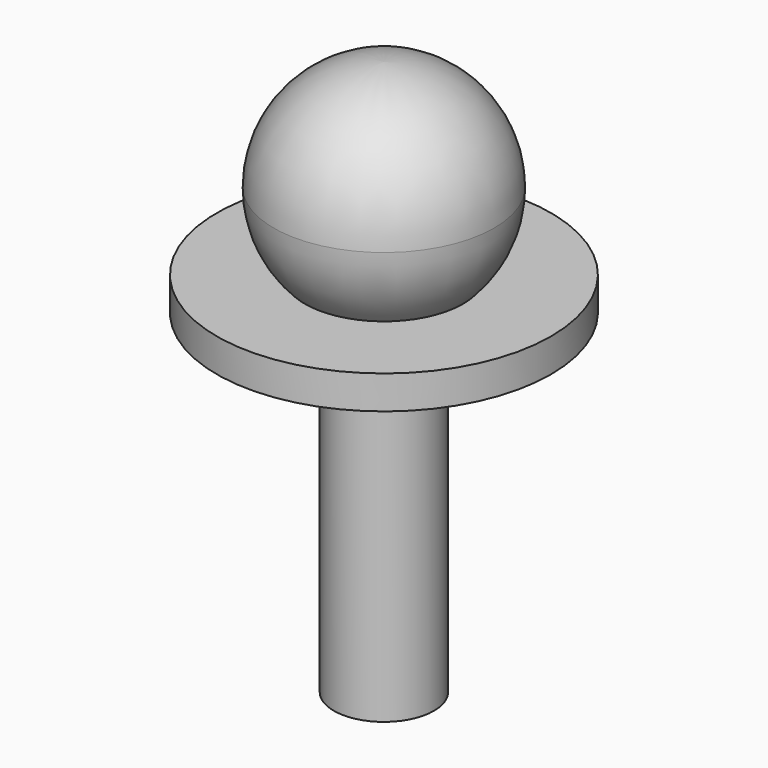
from build123d import *

# Parameters (mm, degrees)
F0_R      = 4.191
F1_DEPTH  = 73.66
F2_R      = 4.191
F3_DEPTH  = 8.382
F4_R      = 4.19099
F5_R      = 6.35
F6_DEPTH  = 1.27
F7_R      = 29.9024876922
F8_DEPTH  = 73.66
F9_R      = 1.905
F10_DEPTH = 12.7


# Not quite as in the source:
# - a fillet or chamfer is up to 0.001 mm smaller than in the source, because OpenCascade refuses the exact size


with BuildPart() as f1:
    # F0 (on Top) → F1 (new body)
    with BuildSketch(Plane.XY):
        Circle(F0_R)
    extrude(amount=F1_DEPTH)



with BuildPart() as f3:
    # F2 (on face) → F3 (new body)
    with BuildSketch(Plane.XY.offset(73.66)):
        Circle(F2_R)
    extrude(amount=F3_DEPTH)

    # F4 (radius 4.191 in the source; OpenCascade refuses exactly that, so slightly less here)
    f4_edges = [f3.edges().sort_by_distance(p)[0] for p in [
        (-4.191, 0, 73.66),
        (-4.191, 0, 82.042),
    ]]
    fillet(f4_edges, radius=F4_R)


with BuildPart() as f1_1:
    add(f1.part)

    add(f3.part)  # F6 merges F3
    # F5 (on face) → F6 (join)
    with BuildSketch(Plane.XY.offset(73.66)):
        Circle(F5_R)
    extrude(amount=F6_DEPTH)

    # F7 (on face) → F8 (cut)
    with BuildSketch(Plane(origin=(0, 0, 0), x_dir=(1, 0, 0), z_dir=(0, 0, -1))):
        Circle(F7_R)
    extrude(amount=-F8_DEPTH, mode=Mode.SUBTRACT)

    # F9 (on face) → F10 (join)
    with BuildSketch(Plane(origin=(0, 0, 73.66), x_dir=(1, 0, 0), z_dir=(0, 0, -1))):
        Circle(F9_R)
    extrude(amount=F10_DEPTH)


solid = f1_1.part
